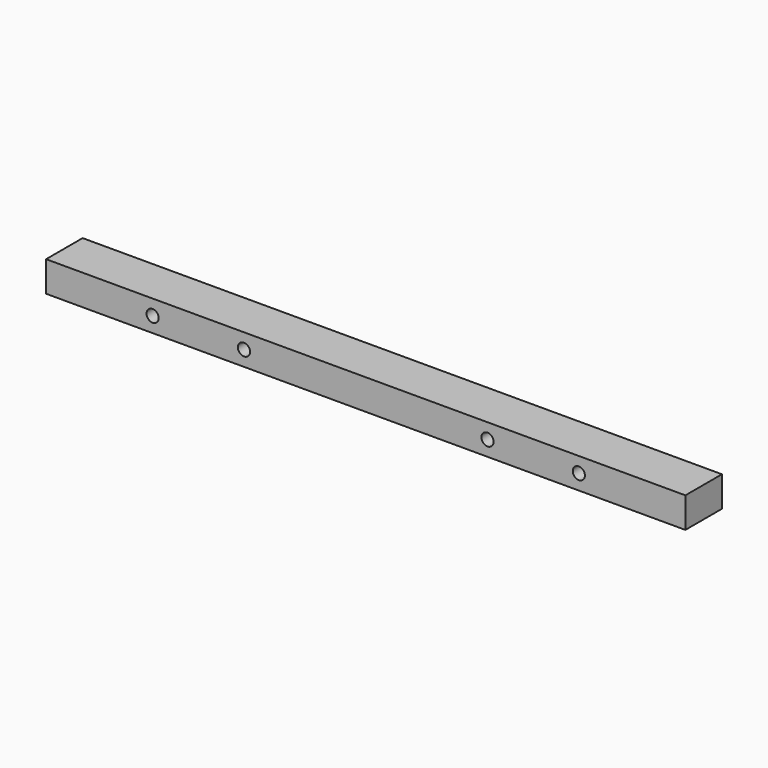
from build123d import *

# Parameters (mm, degrees)
F0_W     = 210
F0_H     = 15
F1_DEPTH = 10
F3_DEPTH = 10


with BuildPart() as f1:
    # F0 (on Top) → F1 (new body)
    with BuildSketch(Plane.XY):
        Rectangle(F0_W, F0_H)
    extrude(amount=F1_DEPTH)

    # F2 (on face) → F3 (cut)
    with BuildSketch(Plane.XZ.offset(7.5)):
        with BuildLine():
            ThreePointArc((68, 5), (70, 3), (72, 5))
            Line((72, 5), (68, 5))
        make_face()
        with BuildLine():
            Line((68, 5), (72, 5))
            ThreePointArc((72, 5), (70, 7), (68, 5))
        make_face()
        with BuildLine():
            ThreePointArc((-72, 5), (-70, 3), (-68, 5))
            Line((-68, 5), (-72, 5))
        make_face()
        with BuildLine():
            Line((-72, 5), (-68, 5))
            ThreePointArc((-68, 5), (-70, 7), (-72, 5))
        make_face()
        with BuildLine():
            ThreePointArc((-42, 5), (-40, 3), (-38, 5))
            Line((-38, 5), (-42, 5))
        make_face()
        with BuildLine():
            Line((-42, 5), (-38, 5))
            ThreePointArc((-38, 5), (-40, 7), (-42, 5))
        make_face()
        with BuildLine():
            ThreePointArc((38, 5), (40, 3), (42, 5))
            Line((42, 5), (38, 5))
        make_face()
        with BuildLine():
            Line((38, 5), (42, 5))
            ThreePointArc((42, 5), (40, 7), (38, 5))
        make_face()
    extrude(amount=-F3_DEPTH, mode=Mode.SUBTRACT)


solid = f1.part
